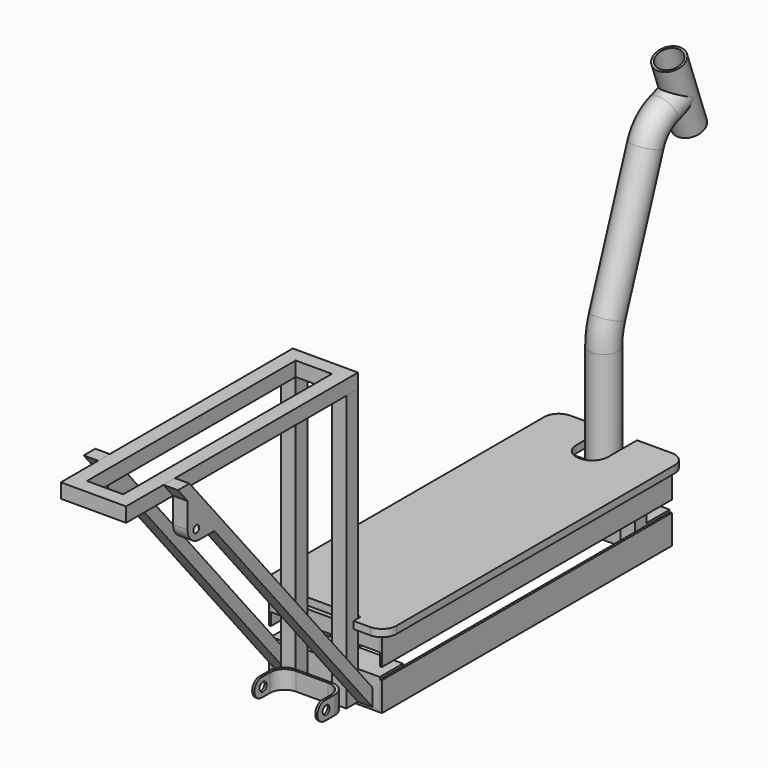
from build123d import *

# Parameters (mm, degrees)
F1_DEPTH  = 500
F2_DEPTH  = 500
F3_W      = 150
F3_H      = 40
F4_DEPTH  = 40
F6_DEPTH  = 20
F8_W      = 150
F8_H      = 20
F9_DEPTH  = 20
F8_H_2    = 40
F10_DEPTH = 40
F11_W     = 20
F11_H     = 380
F12_DEPTH = 20
F13_W     = 90
F13_H     = 400
F13_W_2   = 50
F13_H_2   = 360
F14_DEPTH = 20
F15_R     = 5
F16_DEPTH = 20
F21_R     = 20
F21_R_2   = 17.6
F23_W     = 20
F23_H     = 100
F25_R     = 17
F27_DEPTH = 514.2668195831
F29_DEPTH = 10
F31_DEPTH = 25
F32_R     = 12.49999
F33_R     = 6
F34_DEPTH = 135.001


# Not quite as in the source:
# - a fillet or chamfer is up to 0.001 mm smaller than in the source, because OpenCascade refuses the exact size


with BuildPart() as f1:
    # F0 (on Front) → F1 (new body)
    with BuildSketch(Plane.XZ):
        Polygon((-75, 8), (-75, 45), (-38, 45), (-38, 48), (-78, 48), (-78, 8), align=None)
    extrude(amount=F1_DEPTH)


with BuildPart() as f1b:
    # F0 (on Front) → F1, piece 2 (new body)
    with BuildSketch(Plane.XZ):
        Polygon((78, 8), (78, 48), (38, 48), (38, 45), (75, 45), (75, 8), align=None)
    extrude(amount=F1_DEPTH)


with BuildPart() as f2:
    # F0 (on Front) → F2 (new body)
    with BuildSketch(Plane.XZ):
        Polygon((-78, -48), (-38, -48), (-38, -45), (-75, -45), (-75, -8), (-78, -8), align=None)
    extrude(amount=F2_DEPTH)


with BuildPart() as f2b:
    # F0 (on Front) → F2, piece 2 (new body)
    with BuildSketch(Plane.XZ):
        Polygon((38, -45), (38, -48), (78, -48), (78, -8), (75, -8), (75, -45), align=None)
    extrude(amount=F2_DEPTH)


with BuildPart() as f4:
    # F3 (on Front) → F4 (new body)
    with BuildSketch(Plane.XZ):
        with Locations((0, -25)):
            Rectangle(F3_W, F3_H)
    extrude(amount=F4_DEPTH)


with BuildPart() as f6:
    # F5 (on face) → F6 (new body)
    with BuildSketch(Plane.XZ.offset(40)):
        Polygon((75, -45), (75, 45), (-75, 45), (-75, -45), (-55, -45), (-55, 25), (55, 25), (55, -45), align=None)
    extrude(amount=F6_DEPTH)


with BuildPart() as f9:
    # F8 (on offset) → F9 (new body)
    with BuildSketch(Plane.XZ.offset(500)):
        with Locations((0, 35)):
            Rectangle(F8_W, F8_H)
    extrude(amount=-F9_DEPTH)



with BuildPart() as f10:
    # F8 (on offset) → F10 (new body)
    with BuildSketch(Plane.XZ.offset(500)):
        with Locations((0, -25)):
            Rectangle(F8_W, F8_H_2)
    extrude(amount=-F10_DEPTH)


with BuildPart() as f9_1:
    add(f9.part)

    add(f10.part)  # F12 merges F10
    # F11 (on offset) → F12 (join)
    with BuildSketch(Plane.XZ.offset(500)):
        with Locations((-35, 145)):
            Rectangle(F11_W, F11_H)
        with Locations((35, 145)):
            Rectangle(F11_W, F11_H)
    extrude(amount=F12_DEPTH)


with BuildPart() as f14:
    # F13 (on face) → F14 (new body)
    with BuildSketch(Plane.XY.offset(335)):
        with Locations((0, -700)):
            Rectangle(F13_W, F13_H)
        with Locations((0, -700)):
            Rectangle(F13_W_2, F13_H_2, mode=Mode.SUBTRACT)
    extrude(amount=F14_DEPTH)


with BuildPart() as f16:
    # F15 (on face) → F16 (new body)
    with BuildSketch(Plane(origin=(-45, 0, 0), x_dir=(0, -1, 0), z_dir=(-1, 0, 0))):
        with BuildLine():
            Line((815.6398524709, 355), (500, -21.1649281481))
            Line((500, -21.1649281481), (500, -45))
            Line((500, -45), (772.7073801326, 280))
            Line((772.7073801326, 280), (798.8578598474, 280))
            ThreePointArc((798.8578598474, 280), (812.9999954711, 285.8578643763), (818.8578598474, 300))
            Line((818.8578598474, 300), (818.8578598474, 335))
            Line((818.8578598474, 335), (835.6398524709, 355))
            Line((835.6398524709, 355), (815.6398524709, 355))
        make_face()
        with Locations((803.8578598474, 295)):
            Circle(F15_R, mode=Mode.SUBTRACT)
    extrude(amount=F16_DEPTH)


with BuildPart() as f17_1:
    # F17: instance of F16
    add(f16.part.mirror(Plane.YZ))


with BuildPart() as f22:
    # F22: sweep along a path in F18
    with BuildLine(Plane.YZ) as f22_path:
        Line((-20, -5), (-20, 177.3673019292))
        ThreePointArc((-20, 177.3673019292), (-18.4807753012, 194.7321196958), (-13.9692620786, 211.5693162617))
        Line((-13.9692620786, 211.5693162617), (52.0256693962, 392.8889002872))
        ThreePointArc((52.0256693962, 392.8889002872), (63.6549613762, 411.1432321802), (81.9092932692, 422.7725241602))
        Line((81.9092932692, 422.7725241602), (110, 432.9967052697))
    # F21 (on line) → F22 (sweep)
    with BuildSketch(Plane.XY.offset(-5)):
        with Locations((0, -20)):
            Circle(F21_R)
        with Locations((0, -20)):
            Circle(F21_R_2, mode=Mode.SUBTRACT)
    sweep(path=f22_path.line)

    # F23 (on face) → F26 (revolve)
    with BuildSketch(Plane(origin=(0, 236.2949029628, 86.0043111873), x_dir=(-1, 0, 0), z_dir=(0, 0.9396926208, 0.3420201433))):
        with Locations((-10, 369.2615930007)):
            Rectangle(F23_W, F23_H)
    revolve(axis=Axis((0, 110, 432.9967052697), (0, -0.3420201433, 0.9396926208)))

    # F25 (on line) → F27 (cut, through all)
    with BuildSketch(Plane(origin=(0, -143.395910129, 393.9770251217), x_dir=(1, 0, 0), z_dir=(0, -0.3420201433, 0.9396926208))):
        with Locations((0, 251.4597834823)):
            Circle(F25_R)
    extrude(amount=-F27_DEPTH, mode=Mode.SUBTRACT)


with BuildPart() as f29:
    # F28 (on face) → F29 (new body)
    with BuildSketch(Plane.XY.offset(48)):
        with BuildLine():
            Line((-22, 10), (-70, 10))
            ThreePointArc((-70, 10), (-84.1421356237, 4.1421356237), (-90, -10))
            Line((-90, -10), (-90, -490))
            ThreePointArc((-90, -490), (-84.1421356237, -504.1421356237), (-70, -510))
            Line((-70, -510), (-47, -510))
            Line((-47, -510), (-47, -498))
            Line((-47, -498), (47, -498))
            Line((47, -498), (47, -510))
            Line((47, -510), (70, -510))
            ThreePointArc((70, -510), (84.1421356237, -504.1421356237), (90, -490))
            Line((90, -490), (90, -10))
            ThreePointArc((90, -10), (84.1421356237, 4.1421356237), (70, 10))
            Line((70, 10), (22, 10))
            Line((22, 10), (22, -40))
            ThreePointArc((22, -40), (0, -62), (-22, -40))
            Line((-22, -40), (-22, 10))
        make_face()
    extrude(amount=F29_DEPTH)


with BuildPart() as f31:
    # F30 (on face) → F31 (new body)
    with BuildSketch(Plane(origin=(0, 0, -45), x_dir=(1, 0, 0), z_dir=(0, 0, -1))):
        with BuildLine():
            ThreePointArc((-45, 540), (-39.1421356237, 525.8578643763), (-25, 520))
            Line((-25, 520), (25, 520))
            ThreePointArc((25, 520), (39.1421356237, 525.8578643763), (45, 540))
            Line((45, 540), (45, 570))
            Line((45, 570), (42, 570))
            Line((42, 570), (42, 543))
            ThreePointArc((42, 543), (36.1421356237, 528.8578643763), (22, 523))
            Line((22, 523), (-22, 523))
            ThreePointArc((-22, 523), (-36.1421356237, 528.8578643763), (-42, 543))
            Line((-42, 543), (-42, 570))
            Line((-42, 570), (-45, 570))
            Line((-45, 570), (-45, 540))
        make_face()
    extrude(amount=-F31_DEPTH)

    # F32 (radius 12.5 in the source; OpenCascade refuses exactly that, so slightly less here)
    f32_edges = [f31.edges().sort_by_distance(p)[0] for p in [
        (-43.5, -570, -20),
        (43.5, -570, -20),
        (43.5, -570, -45),
        (-43.5, -570, -45),
    ]]
    fillet(f32_edges, radius=F32_R)

    # F33 (on face) → F34 (cut, through all)
    with BuildSketch(Plane(origin=(-45, 0, 0), x_dir=(0, -1, 0), z_dir=(-1, 0, 0))):
        with Locations((555, -32.5)):
            Circle(F33_R)
    extrude(amount=-F34_DEPTH, mode=Mode.SUBTRACT)


solid = Compound([f1.part, f1b.part, f2.part, f2b.part, f4.part, f6.part, f9_1.part, f14.part, f16.part, f17_1.part, f22.part, f29.part, f31.part])
